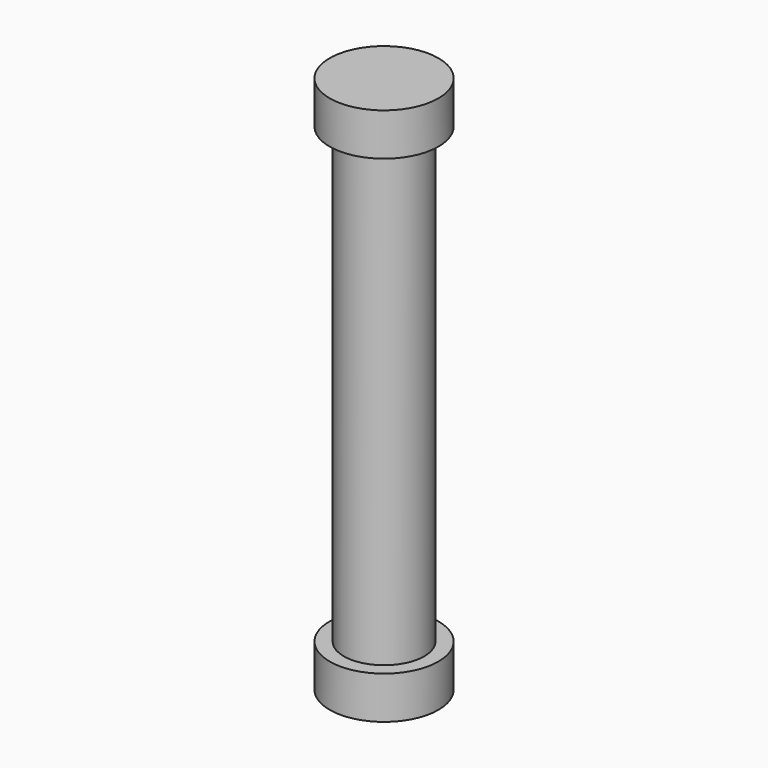
from build123d import *

# Parameters (mm, degrees)
F0_R          = 2.4010472057
F1_DEPTH      = 13.5382
F1_DEPTH_BACK = 13.5382
F2_R          = 3.2490620178
F3_DEPTH      = 2.54


# Not quite as in the source:
# - a pattern or mirror of a feature is missing from the dataset's text; its kind, count and spacing are read off the source's solid


with BuildPart() as f1:
    # F0 (on Top) → F1 (new body, two sides)
    with BuildSketch(Plane.XY) as f1_sk:
        Circle(F0_R)
    extrude(amount=F1_DEPTH)
    extrude(f1_sk.sketch, amount=-F1_DEPTH_BACK)

    # F2 (on face) → F3 (join)
    with BuildSketch(Plane.XY.offset(13.5382)):
        Circle(F2_R)
    f3 = extrude(amount=F3_DEPTH)

    # F3_copies: F3 across plane
    add(f3.mirror(Plane(origin=(0, 0, 0), x_dir=(-1, 0, 0), z_dir=(0, 0, -1))))


solid = f1.part
